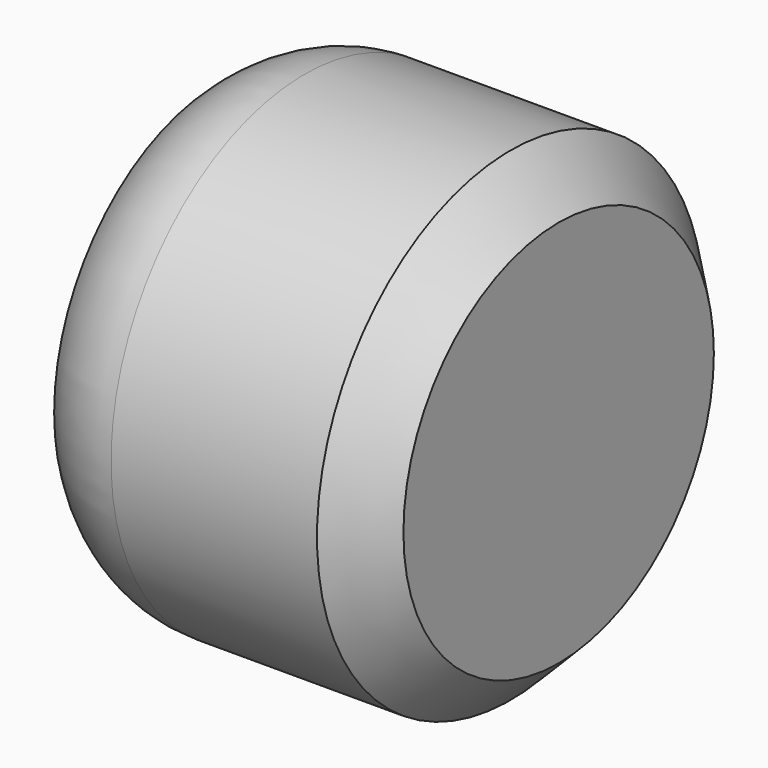
from build123d import *

# Parameters (mm, degrees)
F0_R     = 51.2193764732
F1_DEPTH = 71.882
F2_SIZE  = 10.16
F3_T     = -7.62


# Not quite as in the source:
# - a fillet or chamfer that OpenCascade refuses, or shapes differently, is made with other operations: its cross-section is extruded or revolved along the edge and cut away or added


with BuildPart() as f1:
    # F0 (on Right) → F1 (new body)
    with BuildSketch(Plane.YZ):
        Circle(F0_R)
    extrude(amount=F1_DEPTH)

    # F2
    f2_edges = [f1.edges().sort_by_distance(p)[0] for p in [
        (71.882, -51.219376, 0),
    ]]
    chamfer(f2_edges, length=F2_SIZE)

    # F3
    f3_openings = [f1.faces().sort_by_distance(p)[0] for p in [
        (0, 0, 0),
    ]]
    offset(amount=F3_T, openings=f3_openings)

    # F4: fillet of radius 25.4 on 1 edges, made by hand

    # F4_s1 → F4_t2 (revolve, cut)
    with BuildSketch(Plane.XY):
        with BuildLine():
            ThreePointArc((18.1392282085, 51.2193764732), (8.3018505091, 49.2370193947), (0, 43.5993764732))
            Line((0, 43.5993764732), (0, 51.2193764732))
            Line((0, 51.2193764732), (18.1392282085, 51.2193764732))
        make_face()
    revolve(axis=Axis((0, 0, 0), (1, 0, 0)), mode=Mode.SUBTRACT)


solid = f1.part
